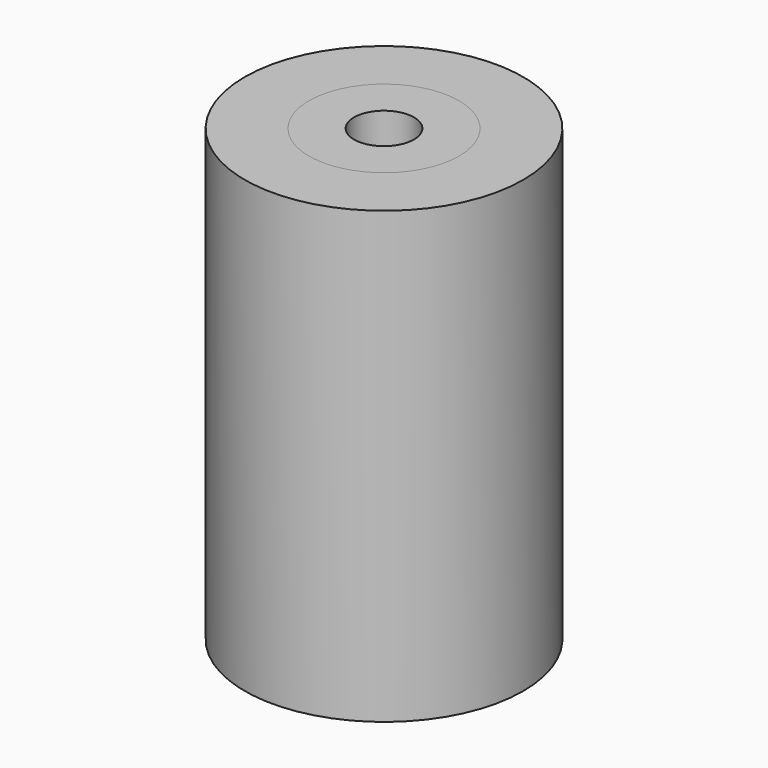
from build123d import *

# Parameters (mm, degrees)
F0_R      = 32.5
F1_DEPTH  = 105
F2_R      = 7
F3_DEPTH  = 110
F4_R      = 25
F5_DEPTH  = 40
F7_DEPTH  = 105
F8_R      = 9
F9_DEPTH  = 105
F10_R     = 17.5
F10_R_2   = 9
F11_DEPTH = 12
F12_R     = 17.5
F13_DEPTH = 12


with BuildPart() as f1:
    # F0 (on Top) → F1 (new body)
    with BuildSketch(Plane.XY):
        Circle(F0_R)
    extrude(amount=F1_DEPTH)

    # F2 (on face) → F3 (cut)
    with BuildSketch(Plane.XY.offset(105)):
        Circle(F2_R)
    extrude(amount=-F3_DEPTH, mode=Mode.SUBTRACT)

    # F4 (on face) → F5 (cut)
    with BuildSketch(Plane(origin=(0, 0, 0), x_dir=(1, 0, 0), z_dir=(0, 0, -1))):
        Circle(F4_R)
    extrude(amount=-F5_DEPTH, mode=Mode.SUBTRACT)


with BuildPart() as f7:
    # F0 (on Top) → F7 (new body)
    with BuildSketch(Plane.XY):
        Circle(F0_R)
    extrude(amount=F7_DEPTH)

    # F8 (on face) → F9 (cut)
    with BuildSketch(Plane(origin=(0, 0, 0), x_dir=(1, 0, 0), z_dir=(0, 0, -1))):
        Circle(F8_R)
    extrude(amount=-F9_DEPTH, mode=Mode.SUBTRACT)

    # F10 (on face) → F11 (cut)
    with BuildSketch(Plane(origin=(0, 0, 0), x_dir=(1, 0, 0), z_dir=(0, 0, -1))):
        Circle(F10_R)
        Circle(F10_R_2, mode=Mode.SUBTRACT)
        Circle(F10_R)
    extrude(amount=-F11_DEPTH, mode=Mode.SUBTRACT)

    # F12 (on face) → F13 (cut)
    with BuildSketch(Plane.XY.offset(105)):
        Circle(F12_R)
    extrude(amount=-F13_DEPTH, mode=Mode.SUBTRACT)


solid = Compound([f1.part, f7.part])
